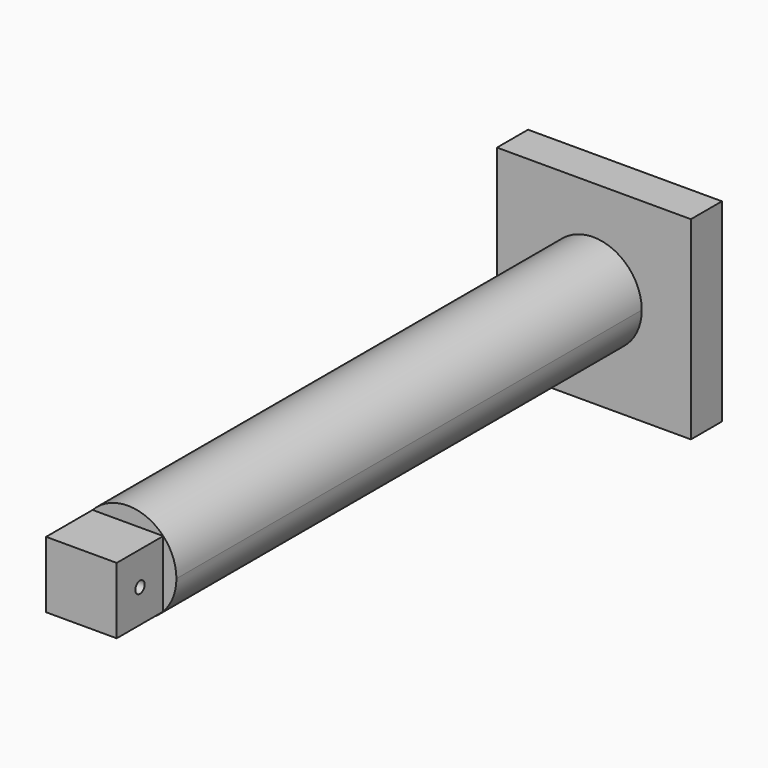
from build123d import *

# Parameters (mm, degrees)
F0_W     = 50
F0_H     = 50
F1_DEPTH = 10
F4_DEPTH = 150
F5_W     = 18.2143148659
F5_H     = 17.1242148423
F6_DEPTH = 15
F8_D     = 3
F8_DEPTH = 50
F8_TIP   = 0.9012909285


with BuildPart() as f1:
    # F0 (on Front) → F1 (new body)
    with BuildSketch(Plane.XZ):
        with Locations((-32.8713305295, -26.3395220041)):
            Rectangle(F0_W, F0_H)
    extrude(amount=F1_DEPTH)

    # F3 (on face) → F4 (join)
    with BuildSketch(Plane.XZ.offset(10)):
        with BuildLine():
            ThreePointArc((-27.7835671151, -31.4272854184), (-26.1262573971, -28.9793373511), (-25.5436490476, -26.0811150074))
            ThreePointArc((-25.5436490476, -26.0811150074), (-36.0539043669, -19.2117363664), (-38.1272124911, -31.5954039658))
            Line((-38.1272124911, -31.5954039658), (-32.8713305295, -26.3395220041))
            Line((-32.8713305295, -26.3395220041), (-27.7835671151, -31.4272854184))
        make_face()
        with BuildLine():
            ThreePointArc((-38.1272124911, -31.5954039658), (-36.0539043669, -19.2117363664), (-25.5436490476, -26.0811150074))
            ThreePointArc((-25.5436490476, -26.0811150074), (-26.1262573971, -28.9793373511), (-27.7835671151, -31.4272854184))
            Line((-27.7835671151, -31.4272854184), (-24.2479633333, -34.9628892003))
            ThreePointArc((-24.2479633333, -34.9628892003), (-21.5068368486, -30.8927638189), (-20.5436490476, -26.0811150074))
            ThreePointArc((-20.5436490476, -26.0811150074), (-37.9675398455, -14.5917590894), (-41.6644969533, -35.1326884279))
            Line((-41.6644969533, -35.1326884279), (-38.1272124911, -31.5954039658))
        make_face()
        with BuildLine():
            Line((-32.8713305295, -26.3395220041), (-38.1272124911, -31.5954039658))
            ThreePointArc((-38.1272124911, -31.5954039658), (-32.921765268, -33.580124565), (-27.7835671151, -31.4272854184))
            Line((-27.7835671151, -31.4272854184), (-32.8713305295, -26.3395220041))
        make_face()
        with BuildLine():
            ThreePointArc((-27.7835671151, -31.4272854184), (-32.921765268, -33.580124565), (-38.1272124911, -31.5954039658))
            Line((-38.1272124911, -31.5954039658), (-41.6644969533, -35.1326884279))
            ThreePointArc((-41.6644969533, -35.1326884279), (-32.9217884335, -38.5805209929), (-24.2479633333, -34.9628892003))
            Line((-24.2479633333, -34.9628892003), (-27.7835671151, -31.4272854184))
        make_face()
    extrude(amount=F4_DEPTH)

    # F5 (on face) → F6 (join)
    with BuildSketch(Plane.XZ.offset(160)):
        with Locations((-33.0436490476, -26.0811150074)):
            Rectangle(F5_W, F5_H)
    extrude(amount=F6_DEPTH)

    # F8
    with Locations(Plane.YZ.offset(-23.9364916147)):
        with Locations((-167.5, -26.0811150074)):
            Hole(F8_D / 2, depth=F8_DEPTH)
            with Locations((0, 0, -(F8_DEPTH + F8_TIP / 2))):  # 118° drill point
                Cone(0, F8_D / 2, F8_TIP, mode=Mode.SUBTRACT)


solid = f1.part
